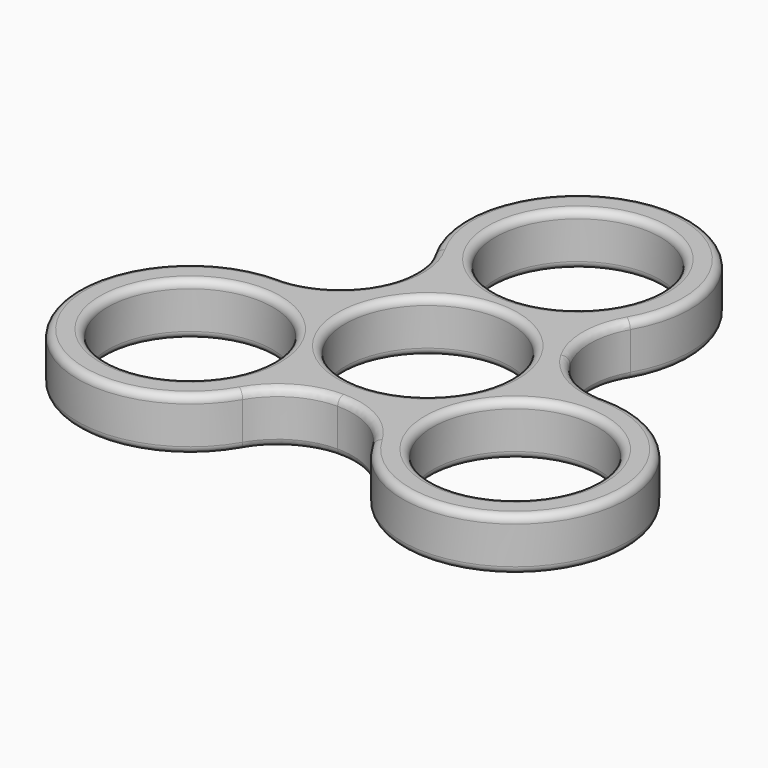
from build123d import *

# Parameters (mm, degrees)
F0_R     = 11
F1_DEPTH = 7
F2_R     = 9.999
F3_R     = 1


# Not quite as in the source:
# - a fillet or chamfer is up to 0.001 mm smaller than in the source, because OpenCascade refuses the exact size


with BuildPart() as f1:
    # F0 (on Top) → F1 (new body)
    with BuildSketch(Plane.XY):
        with BuildLine():
            ThreePointArc((8.2915619759, 12.5), (0, 40), (-8.2915619759, 12.5))
            ThreePointArc((-8.2915619759, 12.5), (-12.9903810568, 7.5), (-14.9710985352, 0.9307033082))
            ThreePointArc((-14.9710985352, 0.9307033082), (-34.6410161514, -20), (-6.6795365594, -13.4307033082))
            ThreePointArc((-6.6795365594, -13.4307033082), (0, -15), (6.6795365594, -13.4307033082))
            ThreePointArc((6.6795365594, -13.4307033082), (34.6410161514, -20), (14.9710985352, 0.9307033082))
            ThreePointArc((14.9710985352, 0.9307033082), (12.9903810568, 7.5), (8.2915619759, 12.5))
        make_face()
        with Locations((-21.6506350946, -12.5)):
            Circle(F0_R, mode=Mode.SUBTRACT)
        Circle(F0_R, mode=Mode.SUBTRACT)
        with Locations((21.6506350946, -12.5)):
            Circle(F0_R, mode=Mode.SUBTRACT)
        with Locations((0, 25)):
            Circle(F0_R, mode=Mode.SUBTRACT)
    extrude(amount=F1_DEPTH)

    # F2 (radius 10 in the source; OpenCascade refuses exactly that, so slightly less here)
    f2_edges = [f1.edges().sort_by_distance(p)[0] for p in [
        (-14.971099, 0.930703, 3.5),
        (-8.291562, 12.5, 3.5),
        (8.291562, 12.5, 3.5),
        (14.971099, 0.930703, 3.5),
        (6.679537, -13.430703, 3.5),
        (-6.679537, -13.430703, 3.5),
    ]]
    fillet(f2_edges, radius=F2_R)

    # F3
    f3_edges = [f1.edges().sort_by_distance(p)[0] for p in [
        (0, 40, 7),
        (-11.65048, 12.5, 7),
        (16.650558, 3.839612, 0),
        (-11, 0, 0),
        (-11, 0, 7),
        (10.650635, -12.5, 7),
        (10.650635, -12.5, 0),
        (-32.650635, -12.5, 0),
        (-32.650635, -12.5, 7),
        (-11, 25, 0),
        (-11, 25, 7),
    ]]
    fillet(f3_edges, radius=F3_R)


solid = f1.part
